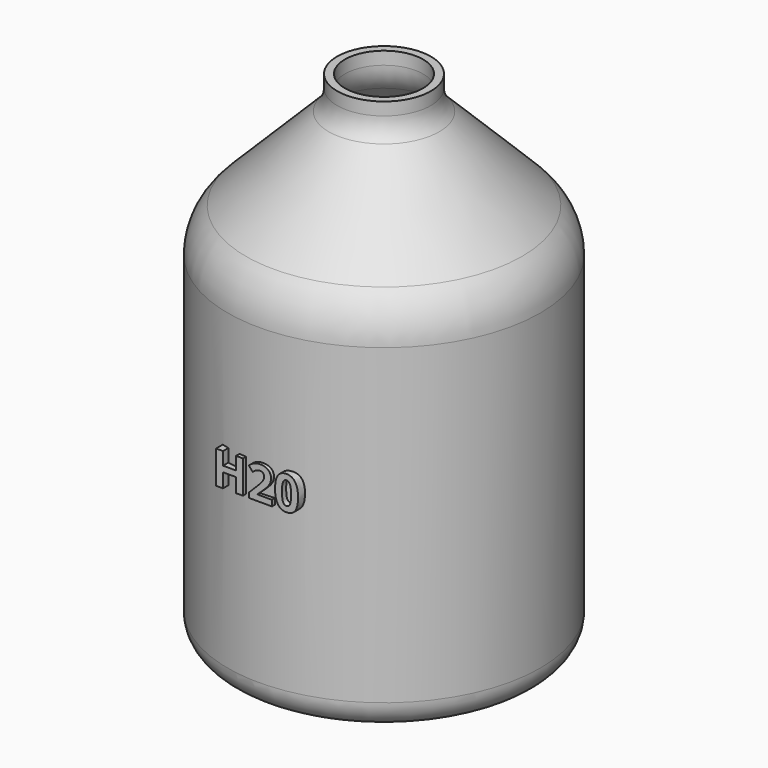
from build123d import *

# Parameters (mm, degrees)
F2_T         = -6.35
F4_TEXT_SIZE = 37.3885863357


# Not quite as in the source:
# - Text() gives the source's letters only with a copy of the font that has no kerning and outlines rounded to 1/6400 em; it was checked with that copy


with BuildPart() as f1:
    # F0 (on Front) → F1 (revolve)
    with BuildSketch(Plane.XZ):
        with BuildLine():
            Line((0, 289.2845715729), (-38.1, 289.2845715729))
            Line((-38.1, 289.2845715729), (-38.1, 278.9030191356))
            ThreePointArc((-38.1, 278.9030191356), (-39.8731858056, 269.9886121084), (-44.9227917574, 262.4313427417))
            Line((-44.9227917574, 262.4313427417), (-112.2161001687, 195.1380343304))
            ThreePointArc((-112.2161001687, 195.1380343304), (-123.1577896169, 178.7626388489), (-127, 159.4465428529))
            Line((-127, 159.4465428529), (-127, -94.5534571471))
            ThreePointArc((-127, -94.5534571471), (-120.391751609, -110.5071800361), (-104.4380287199, -117.1154284271))
            Line((-104.4380287199, -117.1154284271), (0, -117.1154284271))
            Line((0, -117.1154284271), (0, 289.2845715729))
        make_face()
    revolve(axis=Axis((0, 0, 86.0845715729), (0, 0, -1)))

    # F2
    f2_openings = [f1.faces().sort_by_distance(p)[0] for p in [
        (0, 0, 289.284572),
    ]]
    offset(amount=F2_T, openings=f2_openings)

    # F4 (on offset) → F5 (join, up to the next surface of F1)
    with BuildSketch(Plane.XZ.offset(129.54)):
        with Locations((-36.1909831796, 36.5526527166)):
            Text('H20', F4_TEXT_SIZE, font='Open Sans', font_style=FontStyle.BOLD, text_align=(TextAlign.LEFT, TextAlign.BOTTOM))
    extrude(until=Until.NEXT, dir=(0, 1, 0))


solid = f1.part
